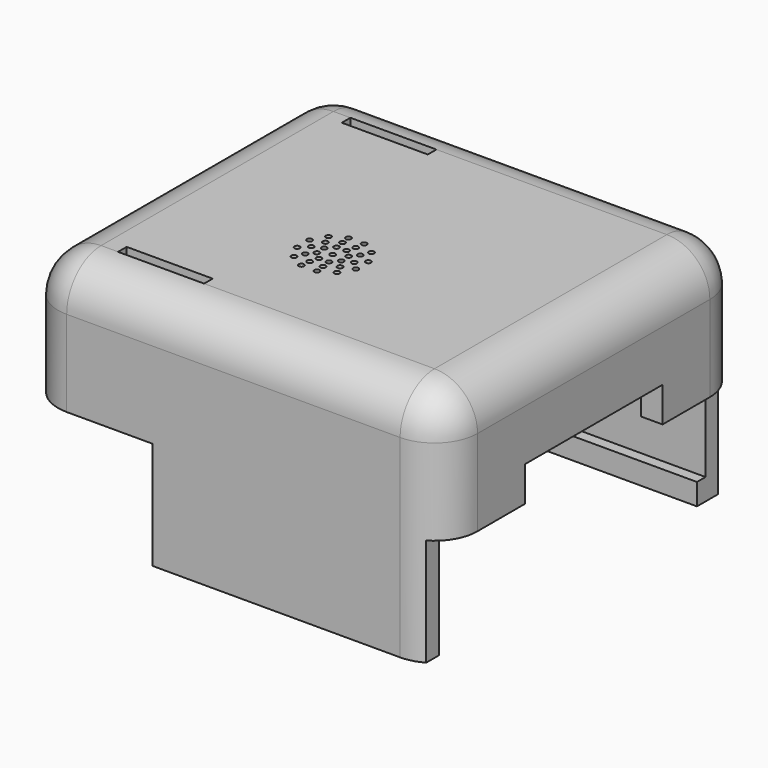
from build123d import *

# Parameters (mm, degrees)
F0_W      = 61.9125
F0_H      = 55.5625
F1_DEPTH  = 19.05
F3_DEPTH  = 58.7375
F4_W      = 3.175
F4_H      = 49.2125
F5_DEPTH  = 15.875
F7_DEPTH  = 15.875
F9_DEPTH  = 15.875
F10_W     = 19.05
F10_H     = 15.875
F10_W_2   = 3.175
F11_DEPTH = 101.6
F12_R     = 6.35
F13_W     = 25.4
F13_H     = 5.1575573161
F14_DEPTH = 25.4
F16_DEPTH = 25.4
F17_W     = 39.6875
F17_H     = 3.175
F18_DEPTH = 1.5875
F19_R     = 0.396875
F20_DEPTH = 25.4


with BuildPart() as f1:
    # F0 (on Top) → F1 (new body)
    with BuildSketch(Plane.XY):
        with Locations((-30.95625, 27.78125)):
            Rectangle(F0_W, F0_H)
    extrude(amount=F1_DEPTH)

    # F2 (on face) → F3 (cut)
    with BuildSketch(Plane.YZ):
        Polygon((27.78125, 15.875), (3.175, 15.875), (3.175, 0), (52.3875, 0), (52.3875, 15.875), align=None)
    extrude(amount=-F3_DEPTH, mode=Mode.SUBTRACT)

    # F4 (on face) → F5 (join)
    with BuildSketch(Plane(origin=(0, 0, 15.875), x_dir=(1, 0, 0), z_dir=(0, 0, -1))):
        with Locations((-1.5875, -27.78125)):
            Rectangle(F4_W, F4_H)
    extrude(amount=F5_DEPTH)

    # F6 (on face) → F7 (join)
    with BuildSketch(Plane(origin=(0, 0, 0), x_dir=(1, 0, 0), z_dir=(0, 0, -1))):
        Polygon((-61.9125, -3.175), (-58.7375, -3.175), (-3.175, -3.175), (0, -3.175), (0, 0), (-61.9125, 0), align=None)
    extrude(amount=F7_DEPTH)

    # F8 (on face) → F9 (join)
    with BuildSketch(Plane(origin=(0, 0, 0), x_dir=(1, 0, 0), z_dir=(0, 0, -1))):
        Polygon((-3.175, -52.3875), (-58.7375, -52.3875), (-61.9125, -52.3875), (-61.9125, -55.5625), (0, -55.5625), (0, -52.3875), align=None)
    extrude(amount=F9_DEPTH)

    # F10 (on face) → F11 (cut)
    with BuildSketch(Plane.XZ):
        with Locations((-52.3875, -7.9375)):
            Rectangle(F10_W, F10_H)
        with Locations((-1.5875, -7.9375)):
            Rectangle(F10_W_2, F10_H)
    extrude(amount=-F11_DEPTH, mode=Mode.SUBTRACT)

    # F12
    f12_edges = [f1.edges().sort_by_distance(p)[0] for p in [
        (-61.9125, 0, 9.525),
        (-30.95625, 0, 19.05),
        (-61.9125, 27.78125, 19.05),
        (0, 0, 9.525),
        (0, 27.78125, 19.05),
        (0, 55.5625, 9.525),
        (-61.9125, 55.5625, 9.525),
        (-30.95625, 55.5625, 19.05),
    ]]
    fillet(f12_edges, radius=F12_R)

    # F13 (on face) → F14 (cut)
    with BuildSketch(Plane.YZ):
        with Locations((27.78125, 2.5787786581)):
            Rectangle(F13_W, F13_H)
    extrude(amount=-F14_DEPTH, mode=Mode.SUBTRACT)

    # F15 (on face) → F16 (cut)
    with BuildSketch(Plane(origin=(0, 0, 15.875), x_dir=(1, 0, 0), z_dir=(0, 0, -1))):
        Polygon((-40.3606608115, -6.35), (-46.7106608115, -6.35), (-53.0606608115, -6.35), (-53.0606608115, -7.9375), (-40.3606608115, -7.9375), align=None)
        Polygon((-40.3606608115, -47.625), (-53.0606608115, -47.625), (-53.0606608115, -49.2125), (-46.7106608115, -49.2125), (-40.3606608115, -49.2125), align=None)
    extrude(amount=-F16_DEPTH, mode=Mode.SUBTRACT)

    # F17 (on face) → F18 (join)
    with BuildSketch(Plane.XZ.offset(-52.3875)):
        with Locations((-23.01875, -14.2875)):
            Rectangle(F17_W, F17_H)
    extrude(amount=F18_DEPTH)

    # F19 (on face) → F20 (cut)
    with BuildSketch(Plane.XY.offset(19.05)):
        with BuildLine():
            Line((-36.4952536137, 24.4581068784), (-36.0983786137, 24.4581068784))
            ThreePointArc((-36.0983786137, 24.4581068784), (-36.7758866175, 24.7387398822), (-36.4952536137, 24.0612318784))
            Line((-36.4952536137, 24.0612318784), (-36.4952536137, 24.4581068784))
        make_face()
        with BuildLine():
            ThreePointArc((-36.4952536137, 24.0612318784), (-36.2146206099, 24.1774738746), (-36.0983786137, 24.4581068784))
            Line((-36.0983786137, 24.4581068784), (-36.4952536137, 24.4581068784))
            Line((-36.4952536137, 24.4581068784), (-36.4952536137, 24.0612318784))
        make_face()
        with Locations((-34.4823842707, 25.6202375354)):
            Circle(F19_R)
        with Locations((-32.1581229567, 25.6202375354)):
            Circle(F19_R)
        with Locations((-30.1452536137, 24.4581068784)):
            Circle(F19_R)
        with Locations((-28.9831229567, 22.4452375354)):
            Circle(F19_R)
        with Locations((-28.9831229567, 20.1209762214)):
            Circle(F19_R)
        with Locations((-30.1452536137, 18.1081068784)):
            Circle(F19_R)
        with Locations((-32.1581229567, 16.9459762214)):
            Circle(F19_R)
        with Locations((-32.3391246566, 18.2635024392)):
            Circle(F19_R)
        with Locations((-30.7516246566, 19.4168887024)):
            Circle(F19_R)
        with BuildLine():
            ThreePointArc((-30.5421286137, 21.2831068784), (-30.1452536137, 20.8862318784), (-29.7483786137, 21.2831068784))
            Line((-29.7483786137, 21.2831068784), (-30.5421286137, 21.2831068784))
        make_face()
        with Locations((-31.5532411462, 20.6476470681)):
            Circle(F19_R)
        with Locations((-32.5201250566, 19.5843024392)):
            Circle(F19_R)
        with BuildLine():
            ThreePointArc((-33.3202536137, 20.8862318784), (-33.0396206099, 21.0024738746), (-32.9233786137, 21.2831068784))
            Line((-32.9233786137, 21.2831068784), (-33.3202536137, 21.2831068784))
            Line((-33.3202536137, 21.2831068784), (-33.3202536137, 20.8862318784))
        make_face()
        with BuildLine():
            Line((-30.5421286137, 21.2831068784), (-29.7483786137, 21.2831068784))
            ThreePointArc((-29.7483786137, 21.2831068784), (-30.1452536137, 21.6799818784), (-30.5421286137, 21.2831068784))
        make_face()
        with Locations((-31.6214491745, 22.0832354355)):
            Circle(F19_R)
        with BuildLine():
            Line((-33.3202536137, 21.2831068784), (-32.9233786137, 21.2831068784))
            ThreePointArc((-32.9233786137, 21.2831068784), (-33.0396206099, 21.5637398822), (-33.3202536137, 21.6799818784))
            Line((-33.3202536137, 21.6799818784), (-33.3202536137, 21.2831068784))
        make_face()
        with Locations((-32.6847938034, 23.0501193459)):
            Circle(F19_R)
        with Locations((-32.3391246566, 24.3027113176)):
            Circle(F19_R)
        with Locations((-30.7516246566, 23.1493250544)):
            Circle(F19_R)
        with BuildLine():
            Line((-34.1203821709, 22.9819113176), (-33.7235071709, 22.9819113176))
            ThreePointArc((-33.7235071709, 22.9819113176), (-34.4010151746, 23.2625443214), (-34.1203821709, 22.5850363176))
            Line((-34.1203821709, 22.5850363176), (-34.1203821709, 22.9819113176))
        make_face()
        with BuildLine():
            ThreePointArc((-34.1203821709, 22.5850363176), (-33.8397491671, 22.7012783139), (-33.7235071709, 22.9819113176))
            Line((-33.7235071709, 22.9819113176), (-34.1203821709, 22.9819113176))
            Line((-34.1203821709, 22.9819113176), (-34.1203821709, 22.5850363176))
        make_face()
        with BuildLine():
            ThreePointArc((-33.9045075709, 24.3027113176), (-33.9125101011, 24.3820080254), (-33.9361949679, 24.4581068784))
            Line((-33.9361949679, 24.4581068784), (-34.6665701738, 24.4581068784))
            ThreePointArc((-34.6665701738, 24.4581068784), (-34.3806792786, 23.9138388478), (-33.9045075709, 24.3027113176))
        make_face()
        with BuildLine():
            Line((-34.6665701738, 24.4581068784), (-33.9361949679, 24.4581068784))
            ThreePointArc((-33.9361949679, 24.4581068784), (-34.3013825709, 24.6995863176), (-34.6665701738, 24.4581068784))
        make_face()
        with Locations((-35.8888825709, 23.1493250544)):
            Circle(F19_R)
        with Locations((-35.0872660812, 21.9185666887)):
            Circle(F19_R)
        with BuildLine():
            Line((-33.7171286137, 21.2831068784), (-33.3202536137, 21.2831068784))
            Line((-33.3202536137, 21.2831068784), (-33.3202536137, 21.6799818784))
            ThreePointArc((-33.3202536137, 21.6799818784), (-33.6008866175, 21.5637398822), (-33.7171286137, 21.2831068784))
        make_face()
        with BuildLine():
            Line((-36.4952536137, 21.2831068784), (-36.0983786137, 21.2831068784))
            ThreePointArc((-36.0983786137, 21.2831068784), (-36.2146206099, 21.5637398822), (-36.4952536137, 21.6799818784))
            Line((-36.4952536137, 21.6799818784), (-36.4952536137, 21.2831068784))
        make_face()
        with BuildLine():
            Line((-36.8921286137, 21.2831068784), (-36.4952536137, 21.2831068784))
            Line((-36.4952536137, 21.2831068784), (-36.4952536137, 21.6799818784))
            ThreePointArc((-36.4952536137, 21.6799818784), (-36.7758866175, 21.5637398822), (-36.8921286137, 21.2831068784))
        make_face()
        with Locations((-37.6573842707, 22.4452375354)):
            Circle(F19_R)
        with Locations((-37.6573842707, 20.1209762214)):
            Circle(F19_R)
        with BuildLine():
            ThreePointArc((-36.8921286137, 21.2831068784), (-36.4952536137, 20.8862318784), (-36.0983786137, 21.2831068784))
            Line((-36.0983786137, 21.2831068784), (-36.4952536137, 21.2831068784))
            Line((-36.4952536137, 21.2831068784), (-36.8921286137, 21.2831068784))
        make_face()
        with Locations((-35.0190580529, 20.4829783213)):
            Circle(F19_R)
        with Locations((-35.8888825709, 19.4168887024)):
            Circle(F19_R)
        with Locations((-36.4952536137, 18.1081068784)):
            Circle(F19_R)
        with Locations((-34.4823842707, 16.9459762214)):
            Circle(F19_R)
        with Locations((-34.3013825709, 18.2635024392)):
            Circle(F19_R)
        with Locations((-33.955713424, 19.5160944109)):
            Circle(F19_R)
        with BuildLine():
            ThreePointArc((-33.7171286137, 21.2831068784), (-33.6008866175, 21.0024738746), (-33.3202536137, 20.8862318784))
            Line((-33.3202536137, 20.8862318784), (-33.3202536137, 21.2831068784))
            Line((-33.3202536137, 21.2831068784), (-33.7171286137, 21.2831068784))
        make_face()
    extrude(amount=-F20_DEPTH, mode=Mode.SUBTRACT)


solid = f1.part
